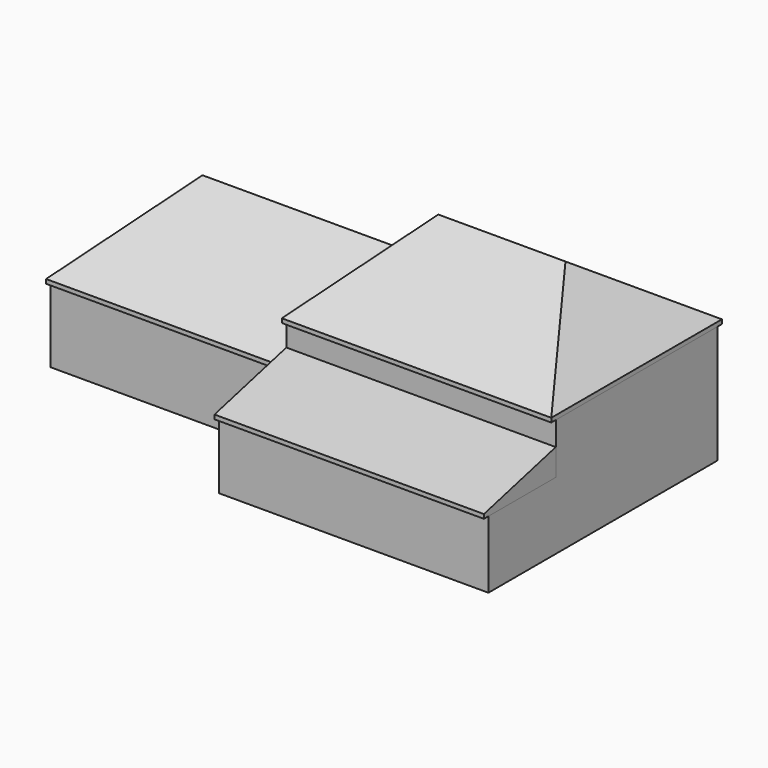
from build123d import *

# Parameters (mm, degrees)
F0_W      = 9753.6
F0_H      = 7315.2
F1_DEPTH  = 4267.2
F3_DEPTH  = 9753.6
F4_W      = 9753.6
F4_H      = 3048
F5_DEPTH  = 2438.4
F7_DEPTH  = 9753.6
F8_W      = 8534.4
F8_H      = 7315.2
F9_DEPTH  = 2743.2
F11_DEPTH = 10972.8
F13_DEPTH = 7721.601
F15_DEPTH = 7721.601


# Not quite as in the source:
# - a feature names something its author has since deleted; it is built from what else it names


with BuildPart() as f1:
    # F0 (on Top) → F1 (new body)
    with BuildSketch(Plane.XY):
        with Locations((4876.8, -3657.6)):
            Rectangle(F0_W, F0_H)
    extrude(amount=F1_DEPTH)

    # F4 (on Top) → F5 (join)
    with BuildSketch(Plane.XY):
        with Locations((4876.8, -8839.2)):
            Rectangle(F4_W, F4_H)
    extrude(amount=F5_DEPTH)


with BuildPart() as f3:
    # F2 (on face) → F3 (new body)
    with BuildSketch(Plane.YZ.offset(9753.6)):
        Polygon((-7518.4, 4419.6), (-7518.4, 4267.2), (-7315.2, 4267.2), (0, 4267.2), (203.2, 4267.2), (203.2, 4419.6), (-3657.6, 6993.4600942352), align=None)
    extrude(amount=-F3_DEPTH)

    # F14 (on face) → F15 (cut, through all)
    with BuildSketch(Plane.XZ.offset(7518.4)):
        Polygon((0, 4419.6), (2573.8600942352, 6993.4600942352), (0, 6993.4600942352), align=None)
        Polygon((7179.7399057648, 6993.4600942352), (9753.6, 4419.6), (9753.6, 6993.4600942352), align=None)
    extrude(amount=-F15_DEPTH, mode=Mode.SUBTRACT)


with BuildPart() as f7:
    # F6 (on face) → F7 (new body, through all)
    with BuildSketch(Plane.YZ.offset(9753.6)):
        Polygon((-10566.4, 2590.8), (-10566.4, 2438.4), (-10363.2, 2438.4), (-7315.2, 2438.4), (-7315.2, 3403.826487487), align=None)
    extrude(amount=-F7_DEPTH)


with BuildPart() as f9:
    # F8 (on Top) → F9 (new body)
    with BuildSketch(Plane.XY):
        with Locations((-4267.2, -3657.6)):
            Rectangle(F8_W, F8_H)
    extrude(amount=F9_DEPTH)


with BuildPart() as f11:
    # F10 (on face) → F11 (new body)
    with BuildSketch(Plane(origin=(-8534.4, 0, 0), x_dir=(0, -1, 0), z_dir=(-1, 0, 0))):
        Polygon((7518.4, 2895.6), (3657.6, 5469.4600942352), (-203.2, 2895.6), (-203.2, 2743.2), (0, 2743.2), (7315.2, 2743.2), (7518.4, 2743.2), align=None)
    extrude(amount=-F11_DEPTH)

    # F12 (on face) → F13 (cut, through all)
    with BuildSketch(Plane.XZ.offset(7518.4)):
        Polygon((-5960.5399057648, 5469.4600942352), (-8534.4, 5469.4600942352), (-8534.4, 2895.6), align=None)
    extrude(amount=-F13_DEPTH, mode=Mode.SUBTRACT)


solid = Compound([f1.part, f3.part, f7.part, f9.part, f11.part])
